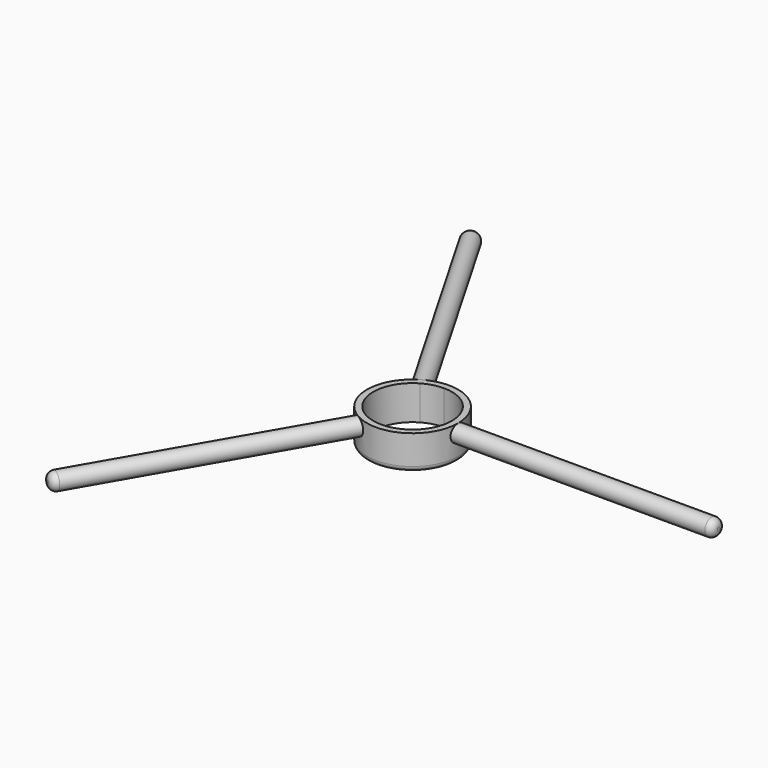
from build123d import *

# Parameters (mm, degrees)
F0_R          = 13.25
F1_DEPTH      = 10
F3_R          = 2.5
F4_DEPTH      = 75
F4_DEPTH_BACK = 2
F5_COUNT      = 3
F6_R          = 1.5
F7_R          = 2
F8_R          = 2


# Not quite as in the source:
# - two fillets or chamfers of one size are made in one step


with BuildPart() as f1:
    # F0 (on Top) → F1 (new body)
    with BuildSketch(Plane.XY):
        Circle(F0_R)
        with BuildLine():
            ThreePointArc((0, 11.43), (8.082230509, 8.082230509), (11.43, 0))
            ThreePointArc((11.43, 0), (8.082230509, -8.082230509), (0, -11.43))
            ThreePointArc((0, -11.43), (-11.43, 0), (0, 11.43))
        make_face(mode=Mode.SUBTRACT)
    extrude(amount=F1_DEPTH)

    # F3 (on offset) → F4 (join, two sides)
    with BuildSketch(Plane.YZ.offset(14)) as f4_sk:
        with Locations((0, 7.5)):
            Circle(F3_R)
    extrude(amount=F4_DEPTH)
    extrude(f4_sk.sketch, amount=-F4_DEPTH_BACK)

    # F5: F1 ×3 about axis
    f5_axis = Axis((0, 0, 10), (0, 0, 1))


with BuildPart() as f1_1:
    add(f1.part)
    for i in range(1, F5_COUNT):
        add(f1.part.rotate(f5_axis, i * 360 / F5_COUNT))

    # F6
    f6_edges = [f1_1.edges().sort_by_distance(p)[0] for p in [
        (-13.25, 0, 0),
    ]]
    fillet(f6_edges, radius=F6_R)

    # F7
    f7_edges = [f1_1.edges().sort_by_distance(p)[0] for p in [
        (89, -2.5, 7.5),
    ]]
    fillet(f7_edges, radius=F7_R)

    # F8
    f8_edges = [f1_1.edges().sort_by_distance(p)[0] for p in [
        (-46.665064, -75.826261, 7.5),
        (-42.334936, 78.326261, 7.5),
    ]]
    fillet(f8_edges, radius=F8_R)


solid = f1_1.part
